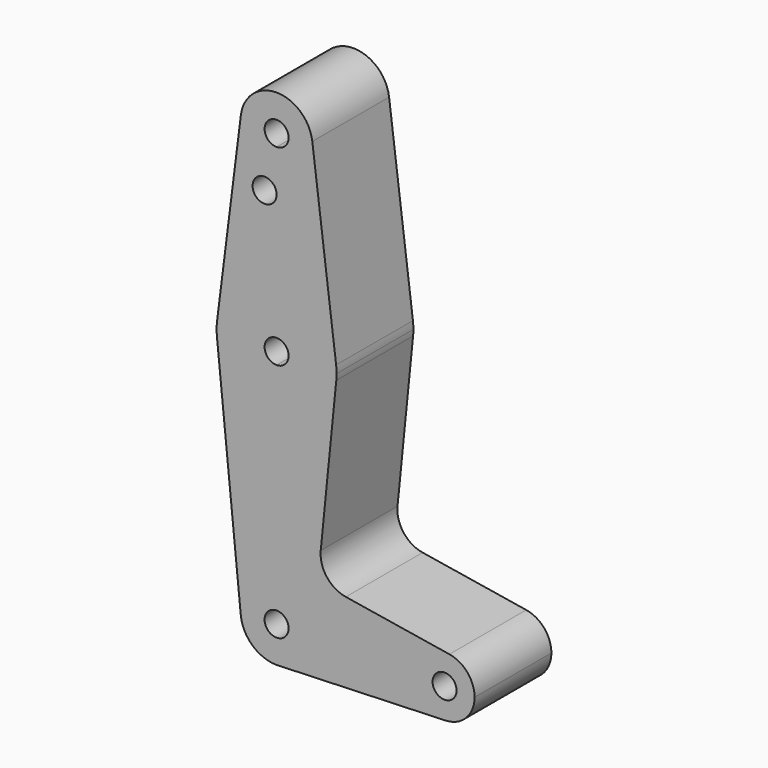
from build123d import *

# Parameters (mm, degrees)
F0_R     = 3.175
F1_DEPTH = 25.4


# Not quite as in the source:
# - a feature of the source that left no trace in its solid (it failed there, or was rolled back) is left out


with BuildPart() as f1:
    # F0 (on Front) → F1 (new body)
    with BuildSketch(Plane.XZ):
        with BuildLine():
            ThreePointArc((9.525, 75.7764706288), (6.7351920908, 69.041278538), (0, 66.2514706288))
            Line((0, 66.2514706288), (0, 61.5016706288))
            Line((0, 61.5016706288), (0, 40.8514706288))
            ThreePointArc((0, 40.8514706288), (10.5003255158, 36.8827206288), (15.7504882737, 26.9608456288))
            Line((15.7504882737, 26.9608456288), (9.4502929642, 76.9670956288))
            ThreePointArc((9.4502929642, 76.9670956288), (9.5063048942, 76.3729538708), (9.525, 75.7764706288))
        make_face()
        with BuildLine():
            ThreePointArc((-9.4502929642, 76.9670956288), (-7.14375, 69.4762753193), (0, 66.2514706288))
            ThreePointArc((0, 66.2514706288), (6.7351920908, 69.041278538), (9.525, 75.7764706288))
            ThreePointArc((9.525, 75.7764706288), (9.5063048942, 76.3729538708), (9.4502929642, 76.9670956288))
            ThreePointArc((9.4502929642, 76.9670956288), (0, 85.3014706288), (-9.4502929642, 76.9670956288))
        make_face()
        with BuildLine():
            ThreePointArc((3.175, 75.7764706288), (2.2450640303, 73.5314065985), (0, 72.6014706288))
            ThreePointArc((0, 72.6014706288), (-2.2450640303, 78.0215346591), (3.175, 75.7764706288))
        make_face(mode=Mode.SUBTRACT)
        with BuildLine():
            Line((0, 61.5016706288), (0, 66.2514706288))
            ThreePointArc((0, 66.2514706288), (-7.14375, 69.4762753193), (-9.4502929642, 76.9670956288))
            Line((-9.4502929642, 76.9670956288), (-15.7504882737, 26.9608456288))
            ThreePointArc((-15.7504882737, 26.9608456288), (-10.5003255158, 36.8827206288), (0, 40.8514706288))
            Line((0, 40.8514706288), (0, 61.5016706288))
        make_face()
        with Locations((-3.175, 61.5016706288)):
            Circle(F0_R, mode=Mode.SUBTRACT)
        with BuildLine():
            Line((0, 28.1514706288), (0, 40.8514706288))
            ThreePointArc((0, 40.8514706288), (-10.5003255158, 36.8827206288), (-15.7504882737, 26.9608456288))
            ThreePointArc((-15.7504882737, 26.9608456288), (-15.8737438155, 25.1761761155), (-15.7954255641, 23.3889706288))
            ThreePointArc((-15.7954255641, 23.3889706288), (-10.6492737428, 13.2032555305), (0, 9.1014706288))
            Line((0, 9.1014706288), (0, 21.8014706288))
            ThreePointArc((0, 21.8014706288), (-3.175, 24.9764706288), (0, 28.1514706288))
        make_face()
        with BuildLine():
            ThreePointArc((15.7504882737, 26.9608456288), (10.5003255158, 36.8827206288), (0, 40.8514706288))
            Line((0, 40.8514706288), (0, 28.1514706288))
            ThreePointArc((0, 28.1514706288), (2.2450640303, 27.2215346591), (3.175, 24.9764706288))
            ThreePointArc((3.175, 24.9764706288), (2.2450640303, 22.7314065985), (0, 21.8014706288))
            Line((0, 21.8014706288), (0, 9.1014706288))
            ThreePointArc((0, 9.1014706288), (10.6492737428, 13.2032555305), (15.7954255641, 23.3889706288))
            ThreePointArc((15.7954255641, 23.3889706288), (15.8550939106, 24.1817240747), (15.875, 24.9764706288))
            ThreePointArc((15.875, 24.9764706288), (15.8438414904, 25.9706093654), (15.7504882737, 26.9608456288))
        make_face()
        with BuildLine():
            ThreePointArc((0, 9.1014706288), (-10.6492737428, 13.2032555305), (-15.7954255641, 23.3889706288))
            Line((-15.7954255641, 23.3889706288), (-9.4772553384, -39.4760293712))
            ThreePointArc((-9.4772553384, -39.4760293712), (-7.063929059, -32.1339651255), (0, -28.9985293712))
            Line((0, -28.9985293712), (0, 9.1014706288))
        make_face()
        with BuildLine():
            ThreePointArc((15.7954255641, 23.3889706288), (10.6492737428, 13.2032555305), (0, 9.1014706288))
            Line((0, 9.1014706288), (0, -28.9985293712))
            ThreePointArc((0, -28.9985293712), (6.7351920908, -31.7883372804), (9.525, -38.5235293712))
            Line((9.525, -38.5235293712), (36.5125, -38.5235293712))
            ThreePointArc((36.5125, -38.5235293712), (39.3067692229, -32.4777801684), (45.7222218075, -30.6886485219))
            Line((45.7222218075, -30.6886485219), (18.312429941, -26.2378680158))
            ThreePointArc((18.312429941, -26.2378680158), (13.2809615783, -23.2323004998), (11.6763381809, -17.5954313572))
            Line((11.6763381809, -17.5954313572), (15.7954255641, 23.3889706288))
        make_face()
        with BuildLine():
            Line((36.5125, -38.5235293712), (9.525, -38.5235293712))
            ThreePointArc((9.525, -38.5235293712), (6.9705567315, -45.0148284595), (0.6773435479, -48.0244151572))
            Line((0.6773435479, -48.0244151572), (44.7324052746, -46.4560039858))
            ThreePointArc((44.7324052746, -46.4560039858), (38.9380895153, -44.2351621551), (36.5125, -38.5235293712))
        make_face()
        with BuildLine():
            ThreePointArc((0, -28.9985293712), (-7.063929059, -32.1339651255), (-9.4772553384, -39.4760293712))
            ThreePointArc((-9.4772553384, -39.4760293712), (-6.3895642457, -45.5874584302), (0, -48.0485293712))
            Line((0, -48.0485293712), (0.6773435479, -48.0244151572))
            ThreePointArc((0.6773435479, -48.0244151572), (6.9705567315, -45.0148284595), (9.525, -38.5235293712))
            Line((9.525, -38.5235293712), (3.175, -38.5235293712))
            ThreePointArc((3.175, -38.5235293712), (-2.2450640303, -40.7685934015), (0, -35.3485293712))
            Line((0, -35.3485293712), (0, -28.9985293712))
        make_face()
        with BuildLine():
            ThreePointArc((9.525, -38.5235293712), (6.7351920908, -31.7883372804), (0, -28.9985293712))
            Line((0, -28.9985293712), (0, -35.3485293712))
            ThreePointArc((0, -35.3485293712), (2.2450640303, -36.2784653409), (3.175, -38.5235293712))
            Line((3.175, -38.5235293712), (9.525, -38.5235293712))
        make_face()
        with BuildLine():
            ThreePointArc((45.7222218075, -30.6886485219), (39.3067692229, -32.4777801684), (36.5125, -38.5235293712))
            ThreePointArc((36.5125, -38.5235293712), (38.9380895153, -44.2351621551), (44.7324052746, -46.4560039858))
            ThreePointArc((44.7324052746, -46.4560039858), (50.1616327839, -44.0354398559), (52.3875, -38.5235293712))
            ThreePointArc((52.3875, -38.5235293712), (50.4957492028, -33.3802985941), (45.7222218075, -30.6886485219))
        make_face()
        with BuildLine():
            ThreePointArc((47.625, -38.5235293712), (44.45, -41.6985293712), (41.275, -38.5235293712))
            ThreePointArc((41.275, -38.5235293712), (44.45, -35.3485293712), (47.625, -38.5235293712))
        make_face(mode=Mode.SUBTRACT)
    extrude(amount=F1_DEPTH)


solid = f1.part
